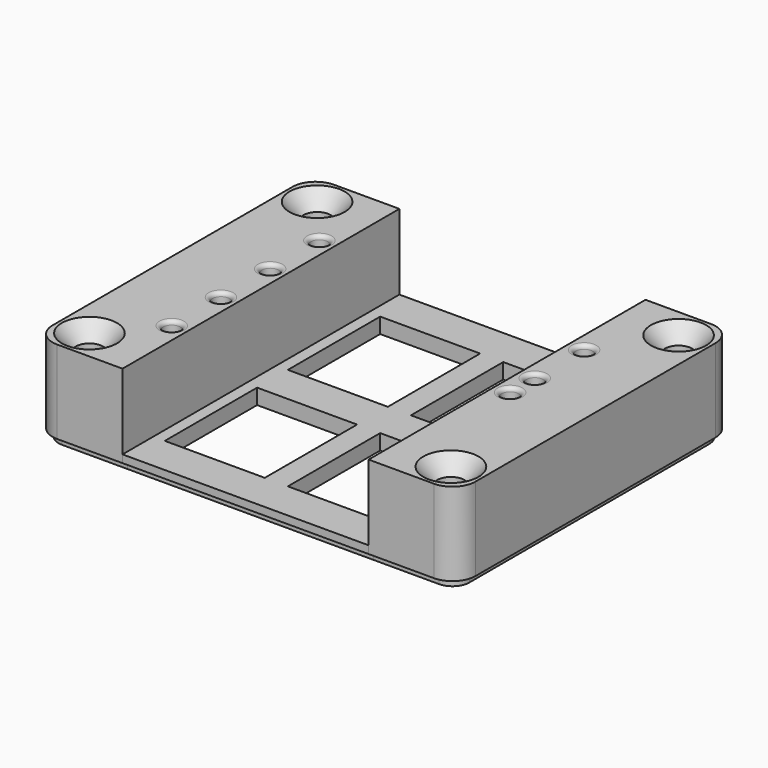
from build123d import *

# Parameters (mm, degrees)
F0_R             = 1.397
F1_DEPTH         = 15
F0_W             = 40.64
F0_H             = 51.3
F0_W_2           = 16.51
F0_H_2           = 19.05
F0_H_3           = 2.925
F2_DEPTH         = 2.54
F3_R             = 3.81
F3_2_R           = 3.81
F4_R             = 0.635
F4_2_R           = 0.635
F7_D             = 4.4958
F7_CSINK_D       = 9.1186
F7_CSINK_ANGLE   = 82
F7_2_D           = 4.4958
F7_2_CSINK_D     = 9.1186
F7_2_CSINK_ANGLE = 82
F9_DEPTH         = 1.27


# Not quite as in the source:
# - a feature names something its author has since deleted; it is built from what else it names


with BuildPart() as f1:
    # F0 (on Top) → F1 (new body)
    with BuildSketch(Plane.XY):
        Polygon((-34.925, -28.575), (-20.32, -28.575), (-20.32, -25.65), (-20.32, 25.65), (-20.32, 28.575), (-34.925, 28.575), align=None)
        with Locations((-22.86, -15.24)):
            Circle(F0_R, mode=Mode.SUBTRACT)
        with Locations((-22.86, -5.08)):
            Circle(F0_R, mode=Mode.SUBTRACT)
        with Locations((-22.86, 5.08)):
            Circle(F0_R, mode=Mode.SUBTRACT)
        with Locations((-22.86, 15.24)):
            Circle(F0_R, mode=Mode.SUBTRACT)
    extrude(amount=F1_DEPTH)

    # F3#2
    f3_2_edges = [f1.edges().sort_by_distance(p)[0] for p in [
        (-34.925, -28.575, 7.5),
        (-34.925, 28.575, 7.5),
    ]]
    fillet(f3_2_edges, radius=F3_2_R)

    # F4
    f4_edges = [f1.edges().sort_by_distance(p)[0] for p in [
        (-24.257, -15.24, 15),
        (-24.257, -5.08, 15),
        (-24.257, 5.08, 15),
        (-24.257, 15.24, 15),
    ]]
    fillet(f4_edges, radius=F4_R)

    # F7 (through all)
    with Locations(Plane.XY.offset(15)):
        with Locations((29.845, -23.495), (29.845, 23.495), (-29.845, 23.495), (-29.845, -23.495)):
            CounterSinkHole(F7_D / 2, F7_CSINK_D / 2, counter_sink_angle=F7_CSINK_ANGLE)


with BuildPart() as f1b:
    # F0 (on Top) → F1, piece 2 (new body)
    with BuildSketch(Plane.XY):
        Polygon((20.32, -28.575), (34.925, -28.575), (34.925, 28.575), (20.32, 28.575), (20.32, 25.65), (20.32, -25.65), align=None)
        with Locations((22.86, -2.54)):
            Circle(F0_R, mode=Mode.SUBTRACT)
        with Locations((22.86, 2.54)):
            Circle(F0_R, mode=Mode.SUBTRACT)
        with Locations((22.8845030069, 12.7)):
            Circle(F0_R, mode=Mode.SUBTRACT)
    extrude(amount=F1_DEPTH)

    # F3
    f3_edges = [f1b.edges().sort_by_distance(p)[0] for p in [
        (34.925, -28.575, 7.5),
        (34.925, 28.575, 7.5),
    ]]
    fillet(f3_edges, radius=F3_R)

    # F4#2
    f4_2_edges = [f1b.edges().sort_by_distance(p)[0] for p in [
        (21.487503, 12.7, 15),
        (21.463, 2.54, 15),
        (21.463, -2.54, 15),
    ]]
    fillet(f4_2_edges, radius=F4_2_R)

    # F7#2 (through all)
    with Locations(Plane.XY.offset(15)):
        with Locations((29.845, -23.495), (29.845, 23.495), (-29.845, 23.495), (-29.845, -23.495)):
            CounterSinkHole(F7_2_D / 2, F7_2_CSINK_D / 2, counter_sink_angle=F7_2_CSINK_ANGLE)


with BuildPart() as f2:
    # F0 (on Top) → F2 (new body)
    with BuildSketch(Plane.XY):
        Rectangle(F0_W, F0_H)
        with Locations((-10.1600003028, -12.7)):
            Rectangle(F0_W_2, F0_H_2, mode=Mode.SUBTRACT)
        with Locations((10.16, -12.7)):
            Rectangle(F0_W_2, F0_H_2, mode=Mode.SUBTRACT)
        with Locations((-10.1600003028, 12.7)):
            Rectangle(F0_W_2, F0_H_2, mode=Mode.SUBTRACT)
        with Locations((10.16, 12.7)):
            Rectangle(F0_W_2, F0_H_2, mode=Mode.SUBTRACT)
        with Locations((0, -27.1125)):
            Rectangle(F0_W, F0_H_3)
        with Locations((0, 27.1125)):
            Rectangle(F0_W, F0_H_3)
    extrude(amount=F2_DEPTH)


with BuildPart() as f9_tool:
    # F8 (on face) → F9 (new body)
    with BuildSketch(Plane.XY):
        with BuildLine():
            Line((20.32, 27.559), (31.115, 27.559))
            ThreePointArc((31.115, 27.559), (33.0906563466, 26.7406563466), (33.909, 24.765))
            Line((33.909, 24.765), (33.909, -24.765))
            ThreePointArc((33.909, -24.765), (33.0906563466, -26.7406563466), (31.115, -27.559))
            Line((31.115, -27.559), (20.32, -27.559))
            Line((20.32, -27.559), (20.32, -28.575))
            Line((20.32, -28.575), (31.115, -28.575))
            ThreePointArc((31.115, -28.575), (33.8090768363, -27.4590768363), (34.925, -24.765))
            Line((34.925, -24.765), (34.925, 24.765))
            ThreePointArc((34.925, 24.765), (33.8090768363, 27.4590768363), (31.115, 28.575))
            Line((31.115, 28.575), (20.32, 28.575))
            Line((20.32, 28.575), (20.32, 27.559))
        make_face()
        with BuildLine():
            Line((-20.32, 27.559), (20.32, 27.559))
            Line((20.32, 27.559), (20.32, 28.575))
            Line((20.32, 28.575), (-20.32, 28.575))
            Line((-20.32, 28.575), (-31.115, 28.575))
            ThreePointArc((-31.115, 28.575), (-33.8090768363, 27.4590768363), (-34.925, 24.765))
            Line((-34.925, 24.765), (-34.925, -24.765))
            ThreePointArc((-34.925, -24.765), (-33.8090768363, -27.4590768363), (-31.115, -28.575))
            Line((-31.115, -28.575), (-20.32, -28.575))
            Line((-20.32, -28.575), (20.32, -28.575))
            Line((20.32, -28.575), (20.32, -27.559))
            Line((20.32, -27.559), (-20.32, -27.559))
            Line((-20.32, -27.559), (-31.115, -27.559))
            ThreePointArc((-31.115, -27.559), (-33.0906563466, -26.7406563466), (-33.909, -24.765))
            Line((-33.909, -24.765), (-33.909, 24.765))
            ThreePointArc((-33.909, 24.765), (-33.0906563466, 26.7406563466), (-31.115, 27.559))
            Line((-31.115, 27.559), (-20.32, 27.559))
        make_face()
    extrude(amount=F9_DEPTH)


with BuildPart() as f1_1:
    add(f1.part)

    # F9: cut by f9_tool
    add(f9_tool.part, mode=Mode.SUBTRACT)


with BuildPart() as f1b_1:
    add(f1b.part)

    # F9: cut by f9_tool
    add(f9_tool.part, mode=Mode.SUBTRACT)


with BuildPart() as f2_1:
    add(f2.part)

    # F9: cut by f9_tool
    add(f9_tool.part, mode=Mode.SUBTRACT)


solid = Compound([f1_1.part, f1b_1.part, f2_1.part])
